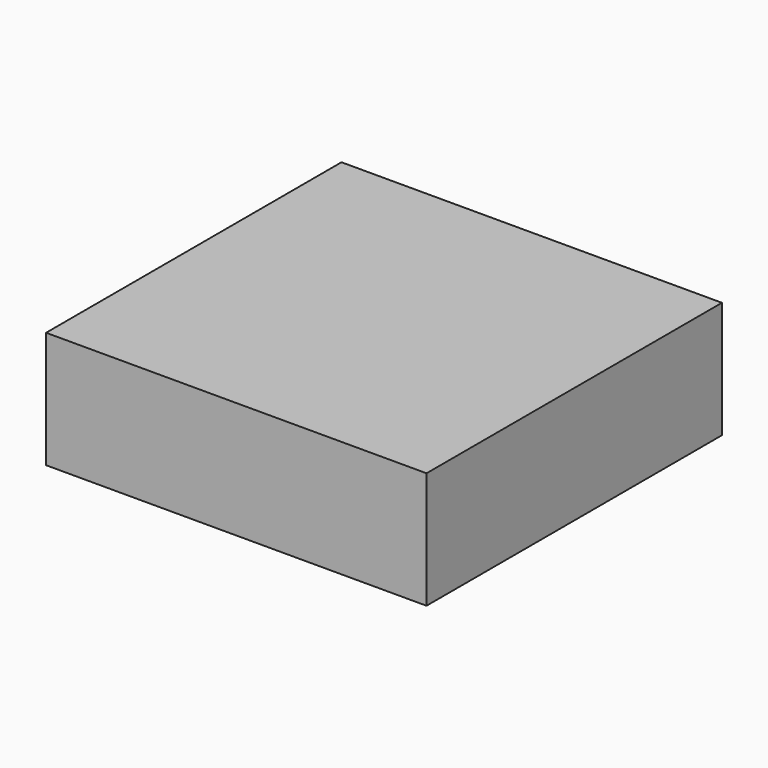
from build123d import *

# Parameters (mm, degrees)
F0_W     = 97.8539548814
F0_H     = 94.975899905
F1_DEPTH = 30


# Not quite as in the source:
# - the program builds the solid bodies; features that only make, move or delete a surface that nothing else refers to are left out


with BuildPart() as f1:
    # F0 (on Top) → F1 (new body)
    with BuildSketch(Plane.XY):
        with Locations((1.2951251119, 3.5975705832)):
            Rectangle(F0_W, F0_H)
    extrude(amount=F1_DEPTH)


solid = f1.part
